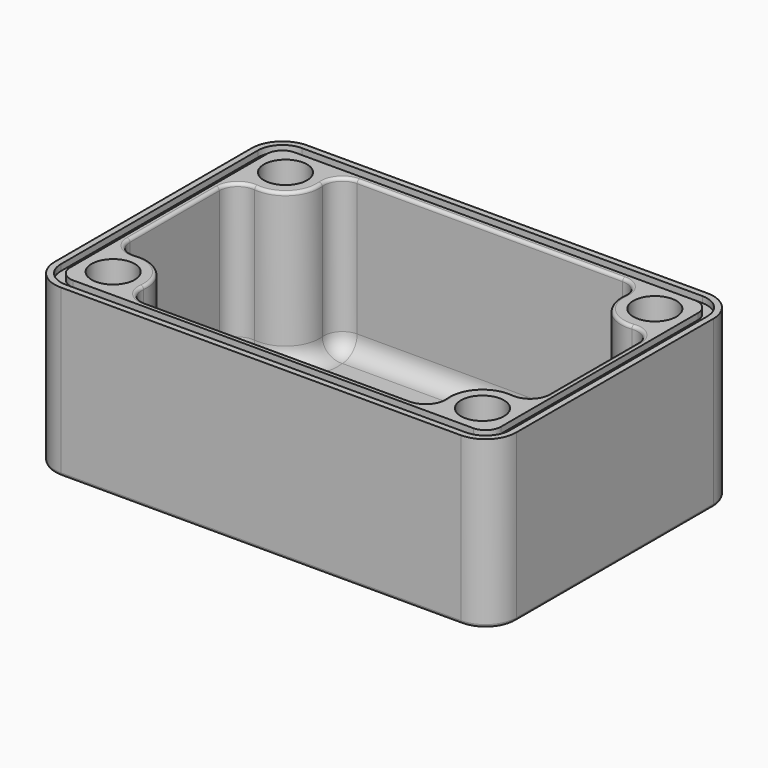
from build123d import *

# Parameters (mm, degrees)
F0_R     = 3.5
F1_DEPTH = 2
F2_DEPTH = 25
F3_DEPTH = 24
F4_R     = 3
F5_R     = 0.5
F6_R     = 0.5


with BuildPart() as f1:
    # F0 (on Top) → F1 (new body)
    with BuildSketch(Plane.XY):
        with BuildLine():
            ThreePointArc((37.5, 20), (36.0355339059, 23.5355339059), (32.5, 25))
            Line((32.5, 25), (-32.5, 25))
            ThreePointArc((-32.5, 25), (-36.0355339059, 23.5355339059), (-37.5, 20))
            Line((-37.5, 20), (-37.5, -20))
            ThreePointArc((-37.5, -20), (-36.0355339059, -23.5355339059), (-32.5, -25))
            Line((-32.5, -25), (32.5, -25))
            ThreePointArc((32.5, -25), (36.0355339059, -23.5355339059), (37.5, -20))
            Line((37.5, -20), (37.5, 20))
        make_face()
        with BuildLine():
            ThreePointArc((32.5, 24), (35.3284271247, 22.8284271247), (36.5, 20))
            Line((36.5, 20), (36.5, -20))
            ThreePointArc((36.5, -20), (35.3284271247, -22.8284271247), (32.5, -24))
            Line((32.5, -24), (-32.5, -24))
            ThreePointArc((-32.5, -24), (-35.3284271247, -22.8284271247), (-36.5, -20))
            Line((-36.5, -20), (-36.5, 20))
            ThreePointArc((-36.5, 20), (-35.3284271247, 22.8284271247), (-32.5, 24))
            Line((-32.5, 24), (32.5, 24))
        make_face(mode=Mode.SUBTRACT)
        with BuildLine():
            Line((36.5, -20), (36.5, 20))
            ThreePointArc((36.5, 20), (35.3284271247, 22.8284271247), (32.5, 24))
            Line((32.5, 24), (-32.5, 24))
            ThreePointArc((-32.5, 24), (-35.3284271247, 22.8284271247), (-36.5, 20))
            Line((-36.5, 20), (-36.5, -20))
            ThreePointArc((-36.5, -20), (-35.3284271247, -22.8284271247), (-32.5, -24))
            Line((-32.5, -24), (32.5, -24))
            ThreePointArc((32.5, -24), (35.3284271247, -22.8284271247), (36.5, -20))
        make_face()
        with BuildLine():
            ThreePointArc((32.5, 22.5), (34.267766953, 21.767766953), (35, 20))
            Line((35, 20), (35, -20))
            ThreePointArc((35, -20), (34.267766953, -21.767766953), (32.5, -22.5))
            Line((32.5, -22.5), (-32.5, -22.5))
            ThreePointArc((-32.5, -22.5), (-34.267766953, -21.767766953), (-35, -20))
            Line((-35, -20), (-35, 20))
            ThreePointArc((-35, 20), (-34.267766953, 21.767766953), (-32.5, 22.5))
            Line((-32.5, 22.5), (32.5, 22.5))
        make_face(mode=Mode.SUBTRACT)
        with BuildLine():
            Line((35, -20), (35, 20))
            ThreePointArc((35, 20), (34.267766953, 21.767766953), (32.5, 22.5))
            Line((32.5, 22.5), (-32.5, 22.5))
            ThreePointArc((-32.5, 22.5), (-34.267766953, 21.767766953), (-35, 20))
            Line((-35, 20), (-35, -20))
            ThreePointArc((-35, -20), (-34.267766953, -21.767766953), (-32.5, -22.5))
            Line((-32.5, -22.5), (32.5, -22.5))
            ThreePointArc((32.5, -22.5), (34.267766953, -21.767766953), (35, -20))
        make_face()
        with BuildLine():
            ThreePointArc((32.5, 21.5), (33.5606601718, 21.0606601718), (34, 20))
            Line((34, 20), (34, 13.7250827824))
            Line((34, 13.7250827824), (34, -13.7250827824))
            Line((34, -13.7250827824), (34, -20))
            ThreePointArc((34, -20), (33.5606601718, -21.0606601718), (32.5, -21.5))
            Line((32.5, -21.5), (26.2250827824, -21.5))
            Line((26.2250827824, -21.5), (-26.2250827824, -21.5))
            Line((-26.2250827824, -21.5), (-32.5, -21.5))
            ThreePointArc((-32.5, -21.5), (-33.5606601718, -21.0606601718), (-34, -20))
            Line((-34, -20), (-34, -13.7250827824))
            Line((-34, -13.7250827824), (-34, 13.7250827824))
            Line((-34, 13.7250827824), (-34, 20))
            ThreePointArc((-34, 20), (-33.5606601718, 21.0606601718), (-32.5, 21.5))
            Line((-32.5, 21.5), (-26.2250827824, 21.5))
            Line((-26.2250827824, 21.5), (26.2250827824, 21.5))
            Line((26.2250827824, 21.5), (32.5, 21.5))
        make_face(mode=Mode.SUBTRACT)
        with BuildLine():
            Line((34, -13.7250827824), (34, 13.7250827824))
            ThreePointArc((34, 13.7250827824), (26.1109127035, 13.6109127035), (26.2250827824, 21.5))
            Line((26.2250827824, 21.5), (-26.2250827824, 21.5))
            ThreePointArc((-26.2250827824, 21.5), (-26.1109127035, 13.6109127035), (-34, 13.7250827824))
            Line((-34, 13.7250827824), (-34, -13.7250827824))
            ThreePointArc((-34, -13.7250827824), (-26.1109127035, -13.6109127035), (-26.2250827824, -21.5))
            Line((-26.2250827824, -21.5), (26.2250827824, -21.5))
            ThreePointArc((26.2250827824, -21.5), (26.1109127035, -13.6109127035), (34, -13.7250827824))
        make_face()
        with BuildLine():
            Line((34, 13.7250827824), (34, 20))
            ThreePointArc((34, 20), (33.5606601718, 21.0606601718), (32.5, 21.5))
            Line((32.5, 21.5), (26.2250827824, 21.5))
            ThreePointArc((26.2250827824, 21.5), (26.1109127035, 13.6109127035), (34, 13.7250827824))
        make_face()
        with Locations((30, 17.5)):
            Circle(F0_R, mode=Mode.SUBTRACT)
        with BuildLine():
            Line((34, -20), (34, -13.7250827824))
            ThreePointArc((34, -13.7250827824), (26.1109127035, -13.6109127035), (26.2250827824, -21.5))
            Line((26.2250827824, -21.5), (32.5, -21.5))
            ThreePointArc((32.5, -21.5), (33.5606601718, -21.0606601718), (34, -20))
        make_face()
        with Locations((30, -17.5)):
            Circle(F0_R, mode=Mode.SUBTRACT)
        with BuildLine():
            Line((-32.5, -21.5), (-26.2250827824, -21.5))
            ThreePointArc((-26.2250827824, -21.5), (-26.1109127035, -13.6109127035), (-34, -13.7250827824))
            Line((-34, -13.7250827824), (-34, -20))
            ThreePointArc((-34, -20), (-33.5606601718, -21.0606601718), (-32.5, -21.5))
        make_face()
        with Locations((-30, -17.5)):
            Circle(F0_R, mode=Mode.SUBTRACT)
        with BuildLine():
            ThreePointArc((-34, 13.7250827824), (-26.1109127035, 13.6109127035), (-26.2250827824, 21.5))
            Line((-26.2250827824, 21.5), (-32.5, 21.5))
            ThreePointArc((-32.5, 21.5), (-33.5606601718, 21.0606601718), (-34, 20))
            Line((-34, 20), (-34, 13.7250827824))
        make_face()
        with Locations((-30, 17.5)):
            Circle(F0_R, mode=Mode.SUBTRACT)
        with Locations((-30, -17.5)):
            Circle(F0_R)
        with Locations((30, 17.5)):
            Circle(F0_R)
        with Locations((30, -17.5)):
            Circle(F0_R)
        with Locations((-30, 17.5)):
            Circle(F0_R)
    extrude(amount=-F1_DEPTH)

    # F0 (on Top) → F2 (join)
    with BuildSketch(Plane.XY):
        with BuildLine():
            ThreePointArc((37.5, 20), (36.0355339059, 23.5355339059), (32.5, 25))
            Line((32.5, 25), (-32.5, 25))
            ThreePointArc((-32.5, 25), (-36.0355339059, 23.5355339059), (-37.5, 20))
            Line((-37.5, 20), (-37.5, -20))
            ThreePointArc((-37.5, -20), (-36.0355339059, -23.5355339059), (-32.5, -25))
            Line((-32.5, -25), (32.5, -25))
            ThreePointArc((32.5, -25), (36.0355339059, -23.5355339059), (37.5, -20))
            Line((37.5, -20), (37.5, 20))
        make_face()
        with BuildLine():
            ThreePointArc((32.5, 24), (35.3284271247, 22.8284271247), (36.5, 20))
            Line((36.5, 20), (36.5, -20))
            ThreePointArc((36.5, -20), (35.3284271247, -22.8284271247), (32.5, -24))
            Line((32.5, -24), (-32.5, -24))
            ThreePointArc((-32.5, -24), (-35.3284271247, -22.8284271247), (-36.5, -20))
            Line((-36.5, -20), (-36.5, 20))
            ThreePointArc((-36.5, 20), (-35.3284271247, 22.8284271247), (-32.5, 24))
            Line((-32.5, 24), (32.5, 24))
        make_face(mode=Mode.SUBTRACT)
        with BuildLine():
            Line((35, -20), (35, 20))
            ThreePointArc((35, 20), (34.267766953, 21.767766953), (32.5, 22.5))
            Line((32.5, 22.5), (-32.5, 22.5))
            ThreePointArc((-32.5, 22.5), (-34.267766953, 21.767766953), (-35, 20))
            Line((-35, 20), (-35, -20))
            ThreePointArc((-35, -20), (-34.267766953, -21.767766953), (-32.5, -22.5))
            Line((-32.5, -22.5), (32.5, -22.5))
            ThreePointArc((32.5, -22.5), (34.267766953, -21.767766953), (35, -20))
        make_face()
        with BuildLine():
            ThreePointArc((32.5, 21.5), (33.5606601718, 21.0606601718), (34, 20))
            Line((34, 20), (34, 13.7250827824))
            Line((34, 13.7250827824), (34, -13.7250827824))
            Line((34, -13.7250827824), (34, -20))
            ThreePointArc((34, -20), (33.5606601718, -21.0606601718), (32.5, -21.5))
            Line((32.5, -21.5), (26.2250827824, -21.5))
            Line((26.2250827824, -21.5), (-26.2250827824, -21.5))
            Line((-26.2250827824, -21.5), (-32.5, -21.5))
            ThreePointArc((-32.5, -21.5), (-33.5606601718, -21.0606601718), (-34, -20))
            Line((-34, -20), (-34, -13.7250827824))
            Line((-34, -13.7250827824), (-34, 13.7250827824))
            Line((-34, 13.7250827824), (-34, 20))
            ThreePointArc((-34, 20), (-33.5606601718, 21.0606601718), (-32.5, 21.5))
            Line((-32.5, 21.5), (-26.2250827824, 21.5))
            Line((-26.2250827824, 21.5), (26.2250827824, 21.5))
            Line((26.2250827824, 21.5), (32.5, 21.5))
        make_face(mode=Mode.SUBTRACT)
        with BuildLine():
            Line((-32.5, -21.5), (-26.2250827824, -21.5))
            ThreePointArc((-26.2250827824, -21.5), (-26.1109127035, -13.6109127035), (-34, -13.7250827824))
            Line((-34, -13.7250827824), (-34, -20))
            ThreePointArc((-34, -20), (-33.5606601718, -21.0606601718), (-32.5, -21.5))
        make_face()
        with Locations((-30, -17.5)):
            Circle(F0_R, mode=Mode.SUBTRACT)
        with BuildLine():
            Line((34, 13.7250827824), (34, 20))
            ThreePointArc((34, 20), (33.5606601718, 21.0606601718), (32.5, 21.5))
            Line((32.5, 21.5), (26.2250827824, 21.5))
            ThreePointArc((26.2250827824, 21.5), (26.1109127035, 13.6109127035), (34, 13.7250827824))
        make_face()
        with Locations((30, 17.5)):
            Circle(F0_R, mode=Mode.SUBTRACT)
        with BuildLine():
            Line((34, -20), (34, -13.7250827824))
            ThreePointArc((34, -13.7250827824), (26.1109127035, -13.6109127035), (26.2250827824, -21.5))
            Line((26.2250827824, -21.5), (32.5, -21.5))
            ThreePointArc((32.5, -21.5), (33.5606601718, -21.0606601718), (34, -20))
        make_face()
        with Locations((30, -17.5)):
            Circle(F0_R, mode=Mode.SUBTRACT)
        with BuildLine():
            ThreePointArc((-34, 13.7250827824), (-26.1109127035, 13.6109127035), (-26.2250827824, 21.5))
            Line((-26.2250827824, 21.5), (-32.5, 21.5))
            ThreePointArc((-32.5, 21.5), (-33.5606601718, 21.0606601718), (-34, 20))
            Line((-34, 20), (-34, 13.7250827824))
        make_face()
        with Locations((-30, 17.5)):
            Circle(F0_R, mode=Mode.SUBTRACT)
    extrude(amount=F2_DEPTH)

    # F0 (on Top) → F3 (join)
    with BuildSketch(Plane.XY):
        with BuildLine():
            Line((36.5, -20), (36.5, 20))
            ThreePointArc((36.5, 20), (35.3284271247, 22.8284271247), (32.5, 24))
            Line((32.5, 24), (-32.5, 24))
            ThreePointArc((-32.5, 24), (-35.3284271247, 22.8284271247), (-36.5, 20))
            Line((-36.5, 20), (-36.5, -20))
            ThreePointArc((-36.5, -20), (-35.3284271247, -22.8284271247), (-32.5, -24))
            Line((-32.5, -24), (32.5, -24))
            ThreePointArc((32.5, -24), (35.3284271247, -22.8284271247), (36.5, -20))
        make_face()
        with BuildLine():
            ThreePointArc((32.5, 22.5), (34.267766953, 21.767766953), (35, 20))
            Line((35, 20), (35, -20))
            ThreePointArc((35, -20), (34.267766953, -21.767766953), (32.5, -22.5))
            Line((32.5, -22.5), (-32.5, -22.5))
            ThreePointArc((-32.5, -22.5), (-34.267766953, -21.767766953), (-35, -20))
            Line((-35, -20), (-35, 20))
            ThreePointArc((-35, 20), (-34.267766953, 21.767766953), (-32.5, 22.5))
            Line((-32.5, 22.5), (32.5, 22.5))
        make_face(mode=Mode.SUBTRACT)
    extrude(amount=F3_DEPTH)

    # F4
    f4_edges = [f1.edges().sort_by_distance(p)[0] for p in [
        (-26.110913, -13.610913, 0),
        (-34, 0, 0),
        (-26.110913, 13.610913, 0),
        (0, 21.5, 0),
        (26.110913, 13.610913, 0),
        (34, 0, 0),
        (26.110913, -13.610913, 0),
        (0, -21.5, 0),
        (-26.225083, 21.5, 12.5),
        (-34, 13.725083, 12.5),
        (26.225083, 21.5, 12.5),
        (34, 13.725083, 12.5),
        (26.225083, -21.5, 12.5),
        (34, -13.725083, 12.5),
        (-26.225083, -21.5, 12.5),
        (-34, -13.725083, 12.5),
    ]]
    fillet(f4_edges, radius=F4_R)

    # F5
    f5_edges = [f1.edges().sort_by_distance(p)[0] for p in [
        (-26.110913, 13.610913, 25),
    ]]
    fillet(f5_edges, radius=F5_R)

    # F6
    f6_edges = [f1.edges().sort_by_distance(p)[0] for p in [
        (36.035534, -23.535534, -2),
        (37.5, 0, -2),
        (36.035534, 23.535534, -2),
        (0, 25, -2),
        (-36.035534, 23.535534, -2),
        (-37.5, 0, -2),
        (-36.035534, -23.535534, -2),
        (0, -25, -2),
    ]]
    fillet(f6_edges, radius=F6_R)


solid = f1.part
